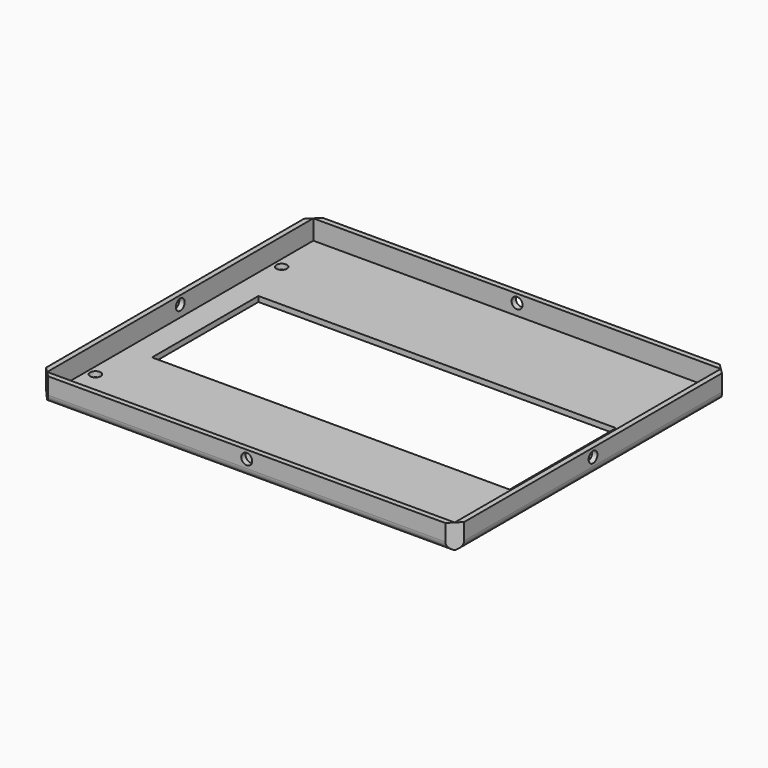
from build123d import *

# Parameters (mm, degrees)
F0_W         = 245
F0_H         = 200
F0_R         = 3.2
F0_W_2       = 215
F0_H_2       = 80
F1_DEPTH     = 3.175
F2_W         = 251.35
F2_H         = 206.35
F2_W_2       = 245
F2_H_2       = 200
F3_DEPTH     = 15
F4_SIZE      = 6.3
F6_R         = 3.3
F7_DEPTH     = 251.351
F8_R         = 3.3
F9_DEPTH     = 206.351
F10_T1_DEPTH = 263.75
F10_T3_DEPTH = 218.75


# Not quite as in the source:
# - a fillet or chamfer that OpenCascade refuses, or shapes differently, is made with other operations: its cross-section is extruded or revolved along the edge and cut away or added


with BuildPart() as f1:
    # F0 (on Top) → F1 (new body)
    with BuildSketch(Plane.XY):
        Rectangle(F0_W, F0_H)
        with Locations((-117.5, -70)):
            Circle(F0_R, mode=Mode.SUBTRACT)
        with Locations((117.5, -70)):
            Circle(F0_R, mode=Mode.SUBTRACT)
        with Locations((-117.5, 70)):
            Circle(F0_R, mode=Mode.SUBTRACT)
        Rectangle(F0_W_2, F0_H_2, mode=Mode.SUBTRACT)
        with Locations((117.5, 70)):
            Circle(F0_R, mode=Mode.SUBTRACT)
    extrude(amount=F1_DEPTH)

    # F2 (on face) → F3 (join)
    with BuildSketch(Plane(origin=(0, 0, 0), x_dir=(1, 0, 0), z_dir=(0, 0, -1))):
        Rectangle(F2_W, F2_H)
        Rectangle(F2_W_2, F2_H_2, mode=Mode.SUBTRACT)
    extrude(amount=-F3_DEPTH)

    # F4
    f4_edges = [f1.edges().sort_by_distance(p)[0] for p in [
        (-125.675, 103.175, 7.5),
        (125.675, 103.175, 7.5),
        (125.675, -103.175, 7.5),
        (-125.675, -103.175, 7.5),
    ]]
    chamfer(f4_edges, length=F4_SIZE)

    # F6 (on face) → F7 (cut, through all)
    with BuildSketch(Plane.YZ.offset(125.675)):
        with Locations((0, 10)):
            Circle(F6_R)
    extrude(amount=-F7_DEPTH, mode=Mode.SUBTRACT)

    # F8 (on face) → F9 (cut, through all)
    with BuildSketch(Plane(origin=(0, 103.175, 0), x_dir=(-1, 0, 0), z_dir=(0, 1, 0))):
        with Locations((0, 10)):
            Circle(F8_R)
    extrude(amount=-F9_DEPTH, mode=Mode.SUBTRACT)

    # F10: fillet of radius 5 on 4 edges, made by hand

    # F10_s2 → F10_t1 (cut)
    with BuildSketch(Plane.YZ.offset(-131.875)):
        with BuildLine():
            ThreePointArc((-98.175, 0), (-101.7105339059, 1.4644660941), (-103.175, 5))
            Line((-103.175, 5), (-103.175, 0))
            Line((-103.175, 0), (-98.175, 0))
        make_face()
        with BuildLine():
            ThreePointArc((98.175, 0), (101.7105339059, 1.4644660941), (103.175, 5))
            Line((103.175, 5), (103.175, 0))
            Line((103.175, 0), (98.175, 0))
        make_face()
    extrude(amount=F10_T1_DEPTH, mode=Mode.SUBTRACT)

    # F10_s4 → F10_t3 (cut)
    with BuildSketch(Plane.XZ.offset(-109.375)):
        with BuildLine():
            ThreePointArc((-120.675, 0), (-124.2105339059, 1.4644660941), (-125.675, 5))
            Line((-125.675, 5), (-125.675, 0))
            Line((-125.675, 0), (-120.675, 0))
        make_face()
        with BuildLine():
            ThreePointArc((120.675, 0), (124.2105339059, 1.4644660941), (125.675, 5))
            Line((125.675, 5), (125.675, 0))
            Line((125.675, 0), (120.675, 0))
        make_face()
    extrude(amount=F10_T3_DEPTH, mode=Mode.SUBTRACT)


solid = f1.part
